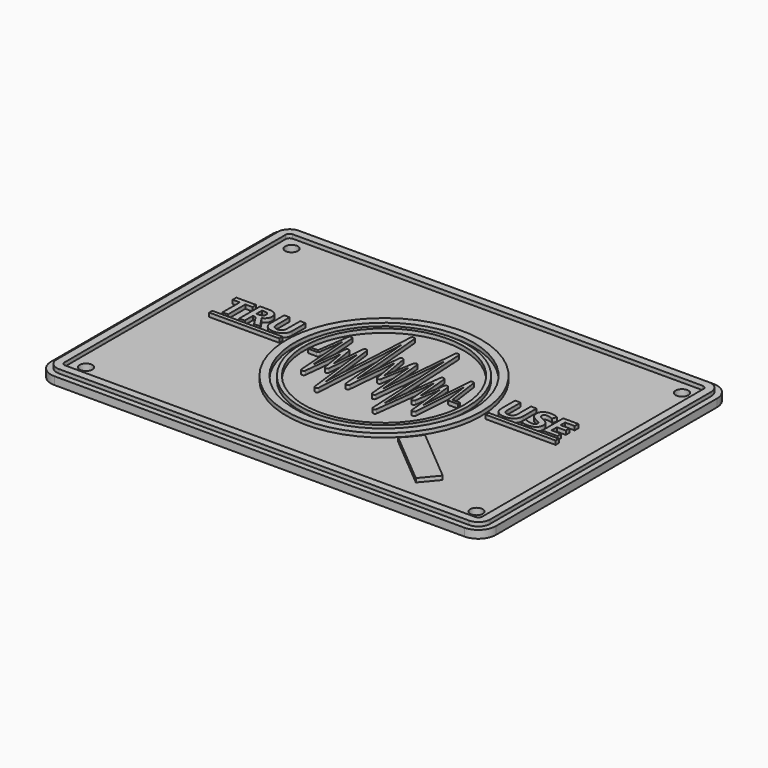
from build123d import *

# Parameters (mm, degrees)
F0_W         = 114.3
F0_H         = 2
F1_DEPTH     = 40
F3_R         = 25
F3_R_2       = 23
F4_DEPTH     = 1.75
F3_W         = 18
F3_H         = 1
F5_R         = 21.5
F5_R_2       = 20.5
F6_DEPTH     = 1.75
F8_DEPTH     = 1.75
F9_TEXT_SIZE = 9.4236111111
F10_DEPTH    = 1.75
F12_DEPTH    = 1.75
F14_DEPTH    = 1.75
F15_R        = 4.5
F16_R        = 1.63195
F17_DEPTH    = 3.0010001


# Not quite as in the source:
# - Text() gives the source's letters only with a copy of the font that has no kerning and outlines rounded to 1/6400 em; it was checked with that copy


with BuildPart() as f1:
    # F0 (on Front) → F1 (new body, symmetric)
    with BuildSketch(Plane.XZ):
        with Locations((0, 1)):
            Rectangle(F0_W, F0_H)
    extrude(amount=F1_DEPTH, both=True)

    # F15
    f15_edges = [f1.edges().sort_by_distance(p)[0] for p in [
        (57.15, 40, 1),
        (57.15, -40, 1),
        (-57.15, -40, 1),
        (-57.15, 40, 1),
    ]]
    fillet(f15_edges, radius=F15_R)

    # F16 (on Top) → F17 (cut, through all)
    with BuildSketch(Plane.XY):
        with Locations((-50.15, 33)):
            Circle(F16_R)
        with Locations((50.15, 33)):
            Circle(F16_R)
        with Locations((-50.15, -33)):
            Circle(F16_R)
        with Locations((50.15, -33)):
            Circle(F16_R)
    extrude(amount=F17_DEPTH, mode=Mode.SUBTRACT)


with BuildPart() as f4:
    # F3 (on offset) → F4 (new body)
    with BuildSketch(Plane.XY.offset(1.25)):
        Circle(F3_R)
        Circle(F3_R_2, mode=Mode.SUBTRACT)
    extrude(amount=F4_DEPTH)


with BuildPart() as f4b:
    # F3 (on offset) → F4, piece 2 (new body)
    with BuildSketch(Plane.XY.offset(1.25)):
        with Locations((-35.495282599, 0)):
            Rectangle(F3_W, F3_H)
    extrude(amount=F4_DEPTH)


with BuildPart() as f4c:
    # F3 (on offset) → F4, piece 3 (new body)
    with BuildSketch(Plane.XY.offset(1.25)):
        with Locations((35.495282599, 0)):
            Rectangle(F3_W, F3_H)
    extrude(amount=F4_DEPTH)


with BuildPart() as f6:
    # F5 (on offset) → F6 (new body)
    with BuildSketch(Plane.XY.offset(1.25)):
        Circle(F5_R)
        Circle(F5_R_2, mode=Mode.SUBTRACT)
    extrude(amount=F6_DEPTH)


with BuildPart() as f8:
    # F7 (on offset) → F8 (new body)
    with BuildSketch(Plane.XY.offset(1.25)):
        with BuildLine():
            ThreePointArc((22.4888517639, -14.9416045437), (20.8499880973, -17.154532822), (18.9942466389, -19.1890227635))
            Line((18.9942466389, -19.1890227635), (32.7830466151, -30.7591997379))
            Line((32.7830466151, -30.7591997379), (36.3183784684, -26.5459553007))
            Line((36.3183784684, -26.5459553007), (22.4888517639, -14.9416045437))
        make_face()
    extrude(amount=F8_DEPTH)


with BuildPart() as f10:
    # F9 (on offset) → F10 (new body)
    with BuildSketch(Plane.XY.offset(1.25)):
        with Locations((-44.4958522604, 1.25)):
            Text('TRU', F9_TEXT_SIZE, font='Open Sans', font_style=FontStyle.BOLD, text_align=(TextAlign.LEFT, TextAlign.BOTTOM))
        with Locations((26.495282599, 1.25)):
            Text('USE', F9_TEXT_SIZE, font='Open Sans', font_style=FontStyle.BOLD, text_align=(TextAlign.LEFT, TextAlign.BOTTOM))
    extrude(amount=F10_DEPTH)


with BuildPart() as f12:
    # F11 (on offset) → F12 (new body)
    with BuildSketch(Plane.XY.offset(1.25)):
        with BuildLine():
            ThreePointArc((55.65, 35.5), (54.7713203436, 37.6213203436), (52.65, 38.5))
            Line((52.65, 38.5), (-52.65, 38.5))
            ThreePointArc((-52.65, 38.5), (-54.7713203436, 37.6213203436), (-55.65, 35.5))
            Line((-55.65, 35.5), (-55.65, -35.5))
            ThreePointArc((-55.65, -35.5), (-54.7713203436, -37.6213203436), (-52.65, -38.5))
            Line((-52.65, -38.5), (52.65, -38.5))
            ThreePointArc((52.65, -38.5), (54.7713203436, -37.6213203436), (55.65, -35.5))
            Line((55.65, -35.5), (55.65, 35.5))
        make_face()
        with BuildLine():
            Line((-52.65, 36.5), (52.65, 36.5))
            ThreePointArc((52.65, 36.5), (53.3571067812, 36.2071067812), (53.65, 35.5))
            Line((53.65, 35.5), (53.65, -35.5))
            ThreePointArc((53.65, -35.5), (53.3571067812, -36.2071067812), (52.65, -36.5))
            Line((52.65, -36.5), (-52.65, -36.5))
            ThreePointArc((-52.65, -36.5), (-53.3571067812, -36.2071067812), (-53.65, -35.5))
            Line((-53.65, -35.5), (-53.65, 35.5))
            ThreePointArc((-53.65, 35.5), (-53.3571067812, 36.2071067812), (-52.65, 36.5))
        make_face(mode=Mode.SUBTRACT)
    extrude(amount=F12_DEPTH)


with BuildPart() as f14:
    # F13 (on offset) → F14 (new body)
    with BuildSketch(Plane.XY.offset(1.25)):
        with BuildLine():
            Line((-19.246, -0.375), (-17.0286783155, -0.375))
            ThreePointArc((-17.0286783155, -0.375), (-16.7006488011, -0.2523547901), (-16.5335442812, 0.0554134495))
            Line((-16.5335442812, 0.0554134495), (-15.6759470089, 6.1575351145))
            Line((-15.6759470089, 6.1575351145), (-14.6795016964, -8.0922967435))
            ThreePointArc((-14.6795016964, -8.0922967435), (-14.1894458745, -8.5573423542), (-13.6834587235, -8.1096827382))
            Line((-13.6834587235, -8.1096827382), (-12.6175820055, 2.0314568202))
            Line((-12.6175820055, 2.0314568202), (-11.5985237765, -4.4026236167))
            ThreePointArc((-11.5985237765, -4.4026236167), (-11.0872298579, -4.8241017977), (-10.6065822572, -4.3679842556))
            Line((-10.6065822572, -4.3679842556), (-9.893414205, 3.7835638814))
            Line((-9.893414205, 3.7835638814), (-7.9235980217, -12.2593015149))
            ThreePointArc((-7.9235980217, -12.2593015149), (-7.4098751976, -12.6980622567), (-6.9280101785, -12.2245348213))
            Line((-6.9280101785, -12.2245348213), (-5.6264531843, 12.6106520923))
            Line((-5.6264531843, 12.6106520923), (-3.8774286777, -7.3807894974))
            ThreePointArc((-3.8774286777, -7.3807894974), (-3.3793313286, -7.837211626), (-2.8812339796, -7.3807894974))
            Line((-2.8812339796, -7.3807894974), (-1.7329588751, 5.7440550049))
            Line((-1.7329588751, 5.7440550049), (-0.4928914516, -1.5313175141))
            ThreePointArc((-0.4928914516, -1.5313175141), (0, -1.9473055091), (0.4928914516, -1.5313175141))
            Line((0.4928914516, -1.5313175141), (1.7329588751, 5.7440550049))
            Line((1.7329588751, 5.7440550049), (2.8812339796, -7.3807894974))
            ThreePointArc((2.8812339796, -7.3807894974), (3.3793313286, -7.837211626), (3.8774286777, -7.3807894974))
            Line((3.8774286777, -7.3807894974), (5.6264531843, 12.6106520923))
            Line((5.6264531843, 12.6106520923), (6.9280101785, -12.2245348213))
            ThreePointArc((6.9280101785, -12.2245348213), (7.4098751976, -12.6980622567), (7.9235980217, -12.2593015149))
            Line((7.9235980217, -12.2593015149), (9.893414205, 3.7835638814))
            Line((9.893414205, 3.7835638814), (10.6065822572, -4.3679842556))
            ThreePointArc((10.6065822572, -4.3679842556), (11.0872298579, -4.8241017977), (11.5985237765, -4.4026236167))
            Line((11.5985237765, -4.4026236167), (12.6175820055, 2.0314568202))
            Line((12.6175820055, 2.0314568202), (13.6834587235, -8.1096827382))
            ThreePointArc((13.6834587235, -8.1096827382), (14.1894458745, -8.5573423542), (14.6795016964, -8.0922967435))
            Line((14.6795016964, -8.0922967435), (15.6759470089, 6.1575351145))
            Line((15.6759470089, 6.1575351145), (16.5335442812, 0.0554134495))
            ThreePointArc((16.5335442812, 0.0554134495), (16.7006488011, -0.2523547901), (17.0286783155, -0.375))
            Line((17.0286783155, -0.375), (19.246, -0.375))
            Line((19.246, -0.375), (19.246, 0.375))
            Line((19.246, 0.375), (17.246, 0.375))
            Line((17.246, 0.375), (16.0876121593, 8.6173577686))
            ThreePointArc((16.0876121593, 8.6173577686), (15.5750283766, 9.0474666316), (15.0936960998, 8.582649455))
            Line((15.0936960998, 8.582649455), (14.1306586945, -5.1894270707))
            Line((14.1306586945, -5.1894270707), (13.1649803009, 3.9983891119))
            ThreePointArc((13.1649803009, 3.9983891119), (12.6808078273, 4.4459535427), (12.1738751829, 4.0243421128))
            Line((12.1738751829, 4.0243421128), (11.1762716402, -2.2742787658))
            Line((11.1762716402, -2.2742787658), (10.4332523534, 6.2184705447))
            ThreePointArc((10.4332523534, 6.2184705447), (9.9438812076, 6.6748165209), (9.4388819285, 6.235827345))
            Line((9.4388819285, 6.235827345), (7.5274316503, -9.3316859008))
            Line((7.5274316503, -9.3316859008), (6.1883155745, 16.2201709822))
            ThreePointArc((6.1883155745, 16.2201709822), (5.6977270103, 16.6939268516), (5.1909034581, 16.2375808754))
            Line((5.1909034581, 16.2375808754), (3.3793313286, -4.4687833146))
            Line((3.3793313286, -4.4687833146), (2.3108705373, 7.7437794136))
            ThreePointArc((2.3108705373, 7.7437794136), (1.8331571313, 8.1997858643), (1.3198817367, 7.7842135473))
            Line((1.3198817367, 7.7842135473), (0, 0.0405770859))
            Line((0, 0.0405770859), (-1.3198817367, 7.7842135473))
            ThreePointArc((-1.3198817367, 7.7842135473), (-1.8331571313, 8.1997858643), (-2.3108705373, 7.7437794136))
            Line((-2.3108705373, 7.7437794136), (-3.3793313286, -4.4687833146))
            Line((-3.3793313286, -4.4687833146), (-5.1909034581, 16.2375808754))
            ThreePointArc((-5.1909034581, 16.2375808754), (-5.6977270103, 16.6939268516), (-6.1883155745, 16.2201709822))
            Line((-6.1883155745, 16.2201709822), (-7.5274316503, -9.3316859008))
            Line((-7.5274316503, -9.3316859008), (-9.4388819285, 6.235827345))
            ThreePointArc((-9.4388819285, 6.235827345), (-9.9438812076, 6.6748165209), (-10.4332523534, 6.2184705447))
            Line((-10.4332523534, 6.2184705447), (-11.1762716402, -2.2742787658))
            Line((-11.1762716402, -2.2742787658), (-12.1738751829, 4.0243421128))
            ThreePointArc((-12.1738751829, 4.0243421128), (-12.6808078273, 4.4459535427), (-13.1649803009, 3.9983891119))
            Line((-13.1649803009, 3.9983891119), (-14.1306586945, -5.1894270707))
            Line((-14.1306586945, -5.1894270707), (-15.0936960998, 8.582649455))
            ThreePointArc((-15.0936960998, 8.582649455), (-15.5750283766, 9.0474666316), (-16.0876121593, 8.6173577686))
            Line((-16.0876121593, 8.6173577686), (-17.246, 0.375))
            Line((-17.246, 0.375), (-19.246, 0.375))
            Line((-19.246, 0.375), (-19.246, -0.375))
        make_face()
    extrude(amount=F14_DEPTH)


with BuildPart() as f1_1:
    add(f1.part)

    # F18: cut F14
    add(f14.part, mode=Mode.SUBTRACT)

    # F19: cut F4, F4b, F4c
    add(f4.part, mode=Mode.SUBTRACT)
    add(f4b.part, mode=Mode.SUBTRACT)
    add(f4c.part, mode=Mode.SUBTRACT)

    # F20: cut F6
    add(f6.part, mode=Mode.SUBTRACT)

    # F21: cut F8
    add(f8.part, mode=Mode.SUBTRACT)

    # F22: cut F10
    add(f10.part, mode=Mode.SUBTRACT)

    # F23: cut F12
    add(f12.part, mode=Mode.SUBTRACT)


solid = Compound([f4.part, f4b.part, f4c.part, f6.part, f8.part, f10.part, f12.part, f14.part, f1_1.part])
